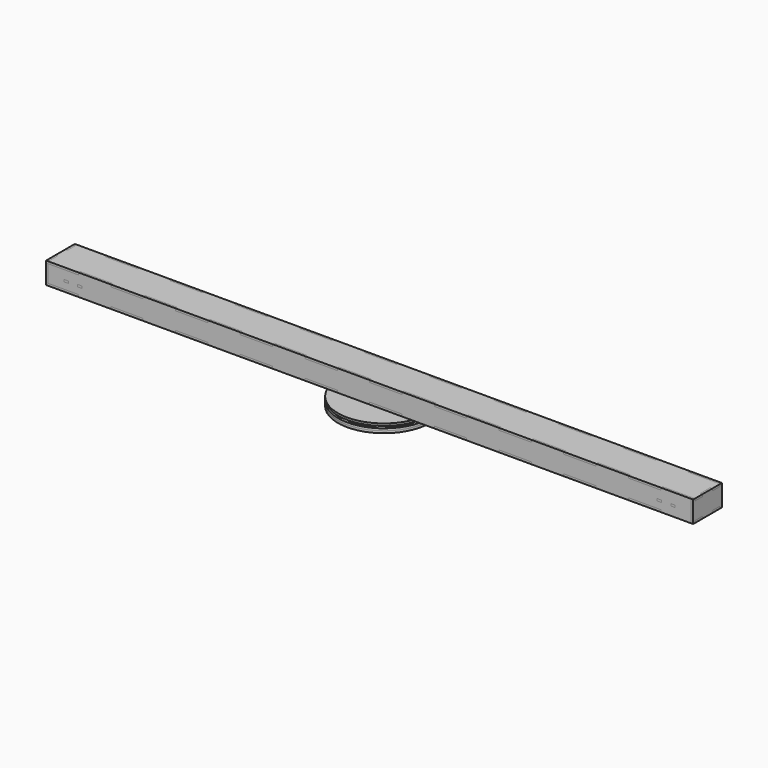
from build123d import *

# Parameters (mm, degrees)
F3_R         = 64
F3_R_2       = 20.5
F3_W         = 6
F3_H         = 6.5
F3_H_2       = 6
F3_R_3       = 1.5
F23_DEPTH    = 3
F5_R         = 20.5
F24_DEPTH    = 3
F6_R         = 1.6
F6_R_2       = 2.5
F6_R_3       = 12.5
F6_W         = 750
F6_H         = 20
F6_W_2       = 3
F6_H_2       = 16.6666666667
F6_W_3       = 45
F6_H_3       = 3
F6_H_4       = 13.6666666667
F25_DEPTH    = 3
F8_W         = 900
F8_H         = 30
F26_DEPTH    = 3
F10_W        = 900
F10_H        = 30
F27_DEPTH    = 3
F12_W        = 50
F12_H        = 30
F28_DEPTH    = 3
F14_W        = 50
F14_H        = 30
F29_DEPTH    = 3
F16_W        = 3
F16_H        = 16.6666666667
F16_W_2      = 45
F16_H_2      = 3
F16_H_3      = 13.6666666667
F30_DEPTH    = 3
F31_DEPTH    = 3
F32_DEPTH    = 3
F33_DEPTH    = 3
F34_DEPTH    = 3
F35_DEPTH    = 3
F18_R        = 1.6
F36_DEPTH    = 3
F37_DEPTH    = 3
F37_FACE_R   = 1.6
F36_FACE_R   = 1.6
F38_DEPTH    = 3
F39_DEPTH    = 3
F21_R        = 64
F40_DEPTH    = 3
F23_FACE_R   = 64
F23_FACE_R_2 = 1.5
F41_DEPTH    = 3
F42_DEPTH    = 3


# Not quite as in the source:
# - a feature names something its author has since deleted; it is built from what else it names


with BuildPart() as f23:
    # F3 (on Top) → F23 (new body)
    with BuildSketch(Plane.XY):
        Circle(F3_R)
        Circle(F3_R_2, mode=Mode.SUBTRACT)
        Circle(F3_R_2)
        with BuildLine():
            ThreePointArc((14.6969384567, 3), (14.9240422951, 1.5076344301), (15, 0))
            ThreePointArc((15, 0), (14.9240422951, -1.5076344301), (14.6969384567, -3))
            ThreePointArc((14.6969384567, -3), (10.6066017178, -10.6066017178), (3, -14.6969384567))
            ThreePointArc((3, -14.6969384567), (0, -15), (-3, -14.6969384567))
            ThreePointArc((-3, -14.6969384567), (-10.6066017178, -10.6066017178), (-14.6969384567, -3))
            ThreePointArc((-14.6969384567, -3), (-15, 0), (-14.6969384567, 3))
            ThreePointArc((-14.6969384567, 3), (-10.6066017178, 10.6066017178), (-3, 14.6969384567))
            ThreePointArc((-3, 14.6969384567), (0, 15), (3, 14.6969384567))
            ThreePointArc((3, 14.6969384567), (10.6066017178, 10.6066017178), (14.6969384567, 3))
        make_face(mode=Mode.SUBTRACT)
        with Locations((0, -6.25)):
            Rectangle(F3_W, F3_H)
        with BuildLine():
            ThreePointArc((-3, -14.6969384567), (0, -15), (3, -14.6969384567))
            Line((3, -14.6969384567), (3, -9.5))
            Line((3, -9.5), (-3, -9.5))
            Line((-3, -9.5), (-3, -14.6969384567))
        make_face()
        with Locations((0, 6.25)):
            Rectangle(F3_W, F3_H)
        with BuildLine():
            Line((3, 9.5), (3, 14.6969384567))
            ThreePointArc((3, 14.6969384567), (0, 15), (-3, 14.6969384567))
            Line((-3, 14.6969384567), (-3, 9.5))
            Line((-3, 9.5), (3, 9.5))
        make_face()
        Rectangle(F3_W, F3_H_2)
        Circle(F3_R_3, mode=Mode.SUBTRACT)
    extrude(amount=-F23_DEPTH)


with BuildPart() as f24:
    # F5 (on offset) → F24 (new body)
    with BuildSketch(Plane.XY.offset(3)):
        Circle(F5_R)
        with BuildLine():
            ThreePointArc((14.6969384567, 3), (14.9240422951, 1.5076344301), (15, 0))
            ThreePointArc((15, 0), (14.9240422951, -1.5076344301), (14.6969384567, -3))
            ThreePointArc((14.6969384567, -3), (10.6066017178, -10.6066017178), (3, -14.6969384567))
            ThreePointArc((3, -14.6969384567), (0, -15), (-3, -14.6969384567))
            ThreePointArc((-3, -14.6969384567), (-10.6066017178, -10.6066017178), (-14.6969384567, -3))
            ThreePointArc((-14.6969384567, -3), (-15, 0), (-14.6969384567, 3))
            ThreePointArc((-14.6969384567, 3), (-10.6066017178, 10.6066017178), (-3, 14.6969384567))
            ThreePointArc((-3, 14.6969384567), (0, 15), (3, 14.6969384567))
            ThreePointArc((3, 14.6969384567), (10.6066017178, 10.6066017178), (14.6969384567, 3))
        make_face(mode=Mode.SUBTRACT)
        with BuildLine():
            ThreePointArc((-3, -14.6969384567), (0, -15), (3, -14.6969384567))
            Line((3, -14.6969384567), (3, -3))
            Line((3, -3), (-3, -3))
            Line((-3, -3), (-3, -14.6969384567))
        make_face()
        with BuildLine():
            ThreePointArc((14.6969384567, -3), (14.9240422951, -1.5076344301), (15, 0))
            ThreePointArc((15, 0), (14.9240422951, 1.5076344301), (14.6969384567, 3))
            Line((14.6969384567, 3), (3, 3))
            Line((3, 3), (-3, 3))
            Line((-3, 3), (-14.6969384567, 3))
            ThreePointArc((-14.6969384567, 3), (-15, 0), (-14.6969384567, -3))
            Line((-14.6969384567, -3), (-3, -3))
            Line((-3, -3), (3, -3))
            Line((3, -3), (14.6969384567, -3))
        make_face()
        with BuildLine():
            Line((3, 3), (3, 14.6969384567))
            ThreePointArc((3, 14.6969384567), (0, 15), (-3, 14.6969384567))
            Line((-3, 14.6969384567), (-3, 3))
            Line((-3, 3), (3, 3))
        make_face()
    extrude(amount=F24_DEPTH)


with BuildPart() as f25:
    # F6 (on offset) → F25 (new body)
    with BuildSketch(Plane.XY.offset(3)):
        Polygon((-360, 22), (-405, 22), (-447, 22), (-447, 8.3333333333), (-447, -8.3333333333), (-447, -22), (-405, -22), (-360, -22), (-315, -22), (-270, -22), (-225, -22), (-180, -22), (-135, -22), (-90, -22), (-45, -22), (0, -22), (45, -22), (90, -22), (135, -22), (180, -22), (225, -22), (270, -22), (315, -22), (360, -22), (405, -22), (447, -22), (447, -8.3333333333), (447, 8.3333333333), (447, 22), (405, 22), (360, 22), (315, 22), (270, 22), (225, 22), (180, 22), (135, 22), (90, 22), (45, 22), (0, 22), (-45, 22), (-90, 22), (-135, 22), (-180, 22), (-225, 22), (-270, 22), (-315, 22), align=None)
        with Locations((-386.593101397, -10.4)):
            Circle(F6_R, mode=Mode.SUBTRACT)
        with Locations((386.593101397, -10.4)):
            Circle(F6_R, mode=Mode.SUBTRACT)
        with Locations((-435.5, 0)):
            Circle(F6_R_2, mode=Mode.SUBTRACT)
        with Locations((-412.5, 0)):
            Circle(F6_R_3, mode=Mode.SUBTRACT)
        with Locations((-386.593101397, 10.4)):
            Circle(F6_R, mode=Mode.SUBTRACT)
        Rectangle(F6_W, F6_H, mode=Mode.SUBTRACT)
        with Locations((412.5, 0)):
            Circle(F6_R_3, mode=Mode.SUBTRACT)
        with Locations((435.5, 0)):
            Circle(F6_R_2, mode=Mode.SUBTRACT)
        with Locations((386.593101397, 10.4)):
            Circle(F6_R, mode=Mode.SUBTRACT)
        with Locations((-448.5, 0)):
            Rectangle(F6_W_2, F6_H_2)
        Polygon((-405, 25), (-450, 25), (-450, 22), (-447, 22), (-405, 22), align=None)
        Polygon((-447, -22), (-450, -22), (-450, -25), (-405, -25), (-405, -22), align=None)
        with Locations((-337.5, -23.5)):
            Rectangle(F6_W_3, F6_H_3)
        with Locations((-337.5, 23.5)):
            Rectangle(F6_W_3, F6_H_3)
        with Locations((-247.5, 23.5)):
            Rectangle(F6_W_3, F6_H_3)
        with Locations((-247.5, -23.5)):
            Rectangle(F6_W_3, F6_H_3)
        with Locations((-157.5, 23.5)):
            Rectangle(F6_W_3, F6_H_3)
        with Locations((-67.5, 23.5)):
            Rectangle(F6_W_3, F6_H_3)
        with Locations((-67.5, -23.5)):
            Rectangle(F6_W_3, F6_H_3)
        with Locations((-157.5, -23.5)):
            Rectangle(F6_W_3, F6_H_3)
        with Locations((22.5, 23.5)):
            Rectangle(F6_W_3, F6_H_3)
        with Locations((22.5, -23.5)):
            Rectangle(F6_W_3, F6_H_3)
        with Locations((112.5, -23.5)):
            Rectangle(F6_W_3, F6_H_3)
        with Locations((112.5, 23.5)):
            Rectangle(F6_W_3, F6_H_3)
        with Locations((202.5, 23.5)):
            Rectangle(F6_W_3, F6_H_3)
        with Locations((202.5, -23.5)):
            Rectangle(F6_W_3, F6_H_3)
        with Locations((292.5, -23.5)):
            Rectangle(F6_W_3, F6_H_3)
        with Locations((292.5, 23.5)):
            Rectangle(F6_W_3, F6_H_3)
        with Locations((382.5, 23.5)):
            Rectangle(F6_W_3, F6_H_3)
        with Locations((382.5, -23.5)):
            Rectangle(F6_W_3, F6_H_3)
        with Locations((448.5, -15.1666666667)):
            Rectangle(F6_W_2, F6_H_4)
        with Locations((448.5, 15.1666666667)):
            Rectangle(F6_W_2, F6_H_4)
        with Locations((412.5, 0)):
            Circle(F6_R_3)
        with Locations((412.5, 0)):
            Circle(F6_R, mode=Mode.SUBTRACT)
        with Locations((-412.5, 0)):
            Circle(F6_R_3)
        with Locations((-412.5, 0)):
            Circle(F6_R, mode=Mode.SUBTRACT)
    extrude(amount=-F25_DEPTH)


with BuildPart() as f26:
    # F8 (on line) → F26 (new body)
    with BuildSketch(Plane(origin=(0, -25, 0), x_dir=(-1, 0, 0), z_dir=(0, 1, 0))):
        with Locations((0, 15)):
            Rectangle(F8_W, F8_H)
    extrude(amount=F26_DEPTH)


with BuildPart() as f27:
    # F10 (on line) → F27 (new body)
    with BuildSketch(Plane(origin=(0, 25, 0), x_dir=(-1, 0, 0), z_dir=(0, 1, 0))):
        with Locations((0, 15)):
            Rectangle(F10_W, F10_H)
    extrude(amount=-F27_DEPTH)


with BuildPart() as f28:
    # F12 (on line) → F28 (new body)
    with BuildSketch(Plane.YZ.offset(450)):
        with Locations((0, 15)):
            Rectangle(F12_W, F12_H)
    extrude(amount=-F28_DEPTH)


with BuildPart() as f29:
    # F14 (on line) → F29 (new body)
    with BuildSketch(Plane.YZ.offset(-450)):
        with Locations((0, 15)):
            Rectangle(F14_W, F14_H)
    extrude(amount=F29_DEPTH)


with BuildPart() as f30:
    # F16 (on line) → F30 (new body)
    with BuildSketch(Plane.XY.offset(30)):
        with Locations((-448.5, 0)):
            Rectangle(F16_W, F16_H)
        Polygon((-405, 25), (-450, 25), (-450, 22), (-447, 22), (-405, 22), align=None)
        Polygon((-447, -22), (-450, -22), (-450, -25), (-405, -25), (-405, -22), align=None)
        with Locations((-337.5, 23.5)):
            Rectangle(F16_W_2, F16_H_2)
        with Locations((-337.5, -23.5)):
            Rectangle(F16_W_2, F16_H_2)
        with Locations((-247.5, 23.5)):
            Rectangle(F16_W_2, F16_H_2)
        with Locations((-247.5, -23.5)):
            Rectangle(F16_W_2, F16_H_2)
        with Locations((-157.5, 23.5)):
            Rectangle(F16_W_2, F16_H_2)
        with Locations((-157.5, -23.5)):
            Rectangle(F16_W_2, F16_H_2)
        with Locations((-67.5, 23.5)):
            Rectangle(F16_W_2, F16_H_2)
        with Locations((-67.5, -23.5)):
            Rectangle(F16_W_2, F16_H_2)
        with Locations((22.5, 23.5)):
            Rectangle(F16_W_2, F16_H_2)
        with Locations((22.5, -23.5)):
            Rectangle(F16_W_2, F16_H_2)
        with Locations((112.5, 23.5)):
            Rectangle(F16_W_2, F16_H_2)
        with Locations((112.5, -23.5)):
            Rectangle(F16_W_2, F16_H_2)
        with Locations((202.5, -23.5)):
            Rectangle(F16_W_2, F16_H_2)
        with Locations((202.5, 23.5)):
            Rectangle(F16_W_2, F16_H_2)
        with Locations((292.5, 23.5)):
            Rectangle(F16_W_2, F16_H_2)
        with Locations((292.5, -23.5)):
            Rectangle(F16_W_2, F16_H_2)
        with Locations((382.5, -23.5)):
            Rectangle(F16_W_2, F16_H_2)
        with Locations((382.5, 23.5)):
            Rectangle(F16_W_2, F16_H_2)
        with Locations((448.5, 15.1666666667)):
            Rectangle(F16_W, F16_H_3)
        with Locations((448.5, -15.1666666667)):
            Rectangle(F16_W, F16_H_3)
        Polygon((-360, 22), (-405, 22), (-447, 22), (-447, 8.3333333333), (-447, -8.3333333333), (-447, -22), (-405, -22), (-360, -22), (-315, -22), (-270, -22), (-225, -22), (-180, -22), (-135, -22), (-90, -22), (-45, -22), (0, -22), (45, -22), (90, -22), (135, -22), (180, -22), (225, -22), (270, -22), (315, -22), (360, -22), (405, -22), (447, -22), (447, -8.3333333333), (447, 8.3333333333), (447, 22), (405, 22), (360, 22), (315, 22), (270, 22), (225, 22), (180, 22), (135, 22), (90, 22), (45, 22), (0, 22), (-45, 22), (-90, 22), (-135, 22), (-180, 22), (-225, 22), (-270, 22), (-315, 22), align=None)
    extrude(amount=-F30_DEPTH)


with BuildPart() as f31_tool:
    # F31 (cut): a face of the model
    f31_faces = [f30.part.faces().sort_by_distance(p)[0] for p in [
        (-1.1003130336, 0, 30),
    ]]
    extrude(f31_faces, amount=-F31_DEPTH)


with BuildPart() as f26_1:
    add(f26.part)

    # F31: cut by f31_tool
    add(f31_tool.part, mode=Mode.SUBTRACT)


with BuildPart() as f27_1:
    add(f27.part)

    # F31: cut by f31_tool
    add(f31_tool.part, mode=Mode.SUBTRACT)


with BuildPart() as f28_1:
    add(f28.part)

    # F31: cut by f31_tool
    add(f31_tool.part, mode=Mode.SUBTRACT)


with BuildPart() as f29_1:
    add(f29.part)

    # F31: cut by f31_tool
    add(f31_tool.part, mode=Mode.SUBTRACT)


with BuildPart() as f32_tool:
    # F32 (cut): a face of the model
    f32_faces = [f25.part.faces().sort_by_distance(p)[0] for p in [
        (446.0986121811, 0, 0),
    ]]
    extrude(f32_faces, amount=-F32_DEPTH)


with BuildPart() as f26_2:
    add(f26_1.part)

    # F32: cut by f32_tool
    add(f32_tool.part, mode=Mode.SUBTRACT)


with BuildPart() as f27_2:
    add(f27_1.part)

    # F32: cut by f32_tool
    add(f32_tool.part, mode=Mode.SUBTRACT)


with BuildPart() as f28_2:
    add(f28_1.part)

    # F32: cut by f32_tool
    add(f32_tool.part, mode=Mode.SUBTRACT)


with BuildPart() as f29_2:
    add(f29_1.part)

    # F32: cut by f32_tool
    add(f32_tool.part, mode=Mode.SUBTRACT)


with BuildPart() as f33_tool:
    # F33 (cut): a face of the model
    f33_faces = [f29_2.part.faces().sort_by_distance(p)[0] for p in [
        (-450, 0, 15),
    ]]
    extrude(f33_faces, amount=-F33_DEPTH)


with BuildPart() as f26_3:
    add(f26_2.part)

    # F33: cut by f33_tool
    add(f33_tool.part, mode=Mode.SUBTRACT)


with BuildPart() as f27_3:
    add(f27_2.part)

    # F33: cut by f33_tool
    add(f33_tool.part, mode=Mode.SUBTRACT)


with BuildPart() as f34_tool:
    # F34 (cut): a face of the model
    f34_faces = [f28_2.part.faces().sort_by_distance(p)[0] for p in [
        (450, 0, 15),
    ]]
    extrude(f34_faces, amount=-F34_DEPTH)


with BuildPart() as f26_4:
    add(f26_3.part)

    # F34: cut by f34_tool
    add(f34_tool.part, mode=Mode.SUBTRACT)


with BuildPart() as f27_4:
    add(f27_3.part)

    # F34: cut by f34_tool
    add(f34_tool.part, mode=Mode.SUBTRACT)


with BuildPart() as f35:
    # F6 (on offset) → F35 (new body)
    with BuildSketch(Plane.XY.offset(3)):
        with Locations((-412.5, 0)):
            Circle(F6_R_3)
        with Locations((-412.5, 0)):
            Circle(F6_R, mode=Mode.SUBTRACT)
    extrude(amount=F35_DEPTH)


with BuildPart() as f36:
    # F18 (on offset) → F36 (new body)
    with BuildSketch(Plane.XY.offset(12)):
        Polygon((-419, 25), (-425, 25), (-425, 22), (-425, -25), (-419, -25), (-419, -22), (-406, -22), (-406, -25), (-400, -25), (-400, 22), (-400, 25), (-406, 25), (-406, 22), (-419, 22), align=None)
        with Locations((-412.5, 0)):
            Circle(F18_R, mode=Mode.SUBTRACT)
    extrude(amount=F36_DEPTH)


with BuildPart() as f37:
    # F18 (on offset) → F37 (new body)
    with BuildSketch(Plane.XY.offset(12)):
        Polygon((406, 25), (400, 25), (400, 22), (400, -25), (406, -25), (406, -22), (419, -22), (419, -25), (425, -25), (425, 22), (425, 25), (419, 25), (419, 22), (406, 22), align=None)
        with Locations((412.5, 0)):
            Circle(F18_R, mode=Mode.SUBTRACT)
    extrude(amount=F37_DEPTH)


with BuildPart() as f37b:
    # F18 (on offset) → F37, piece 2 (new body)
    with BuildSketch(Plane.XY.offset(12)):
        Polygon((-419, 25), (-425, 25), (-425, 22), (-425, -25), (-419, -25), (-419, -22), (-406, -22), (-406, -25), (-400, -25), (-400, 22), (-400, 25), (-406, 25), (-406, 22), (-419, 22), align=None)
        with Locations((-412.5, 0)):
            Circle(F18_R, mode=Mode.SUBTRACT)
    extrude(amount=F37_DEPTH)


with BuildPart() as f38_tool:
    # F37_face (on face) + F36_face (on face) → F38 (new body)
    with BuildSketch(Plane(origin=(412.5, 0, 15), x_dir=(1, 0, 0), z_dir=(0, 0, 1))):
        Polygon((-6.5, 25), (-12.5, 25), (-12.5, -25), (-6.5, -25), (-6.5, -22), (6.5, -22), (6.5, -25), (12.5, -25), (12.5, 25), (6.5, 25), (6.5, 22), (-6.5, 22), align=None)
        Circle(F37_FACE_R, mode=Mode.SUBTRACT)
    with BuildSketch(Plane(origin=(-412.5, 0, 15), x_dir=(1, 0, 0), z_dir=(0, 0, 1))):
        Polygon((-6.5, 25), (-12.5, 25), (-12.5, -25), (-6.5, -25), (-6.5, -22), (6.5, -22), (6.5, -25), (12.5, -25), (12.5, 25), (6.5, 25), (6.5, 22), (-6.5, 22), align=None)
        Circle(F36_FACE_R, mode=Mode.SUBTRACT)
    extrude(amount=-F38_DEPTH)


with BuildPart() as f26_5:
    add(f26_4.part)

    # F38: cut by f38_tool
    add(f38_tool.part, mode=Mode.SUBTRACT)


with BuildPart() as f27_5:
    add(f27_4.part)

    # F38: cut by f38_tool
    add(f38_tool.part, mode=Mode.SUBTRACT)


with BuildPart() as f39:
    # F3 (on Top) → F39 (new body)
    with BuildSketch(Plane.XY):
        with Locations((0, -6.25)):
            Rectangle(F3_W, F3_H)
        Rectangle(F3_W, F3_H_2)
        Circle(F3_R_3, mode=Mode.SUBTRACT)
        with Locations((0, 6.25)):
            Rectangle(F3_W, F3_H)
    extrude(amount=F39_DEPTH)


with BuildPart() as f40:
    # F21 (on offset) → F40 (new body)
    with BuildSketch(Plane.XY.offset(-9)):
        Circle(F21_R)
        with BuildLine():
            ThreePointArc((60.0732729337, 10.5925388377), (60.7678765836, 5.3165003076), (61, 0))
            ThreePointArc((61, 0), (60.7678765836, -5.3165003076), (60.0732729337, -10.5925388377))
            ThreePointArc((60.0732729337, -10.5925388377), (58.9214754036, -15.7879617513), (57.3212498679, -20.8632287429))
            ThreePointArc((57.3212498679, -20.8632287429), (55.2847750092, -25.7797139662), (52.8275496309, -30.5))
            ThreePointArc((52.8275496309, -30.5), (49.9682747016, -34.9881626174), (46.7287110303, -39.2100441909))
            ThreePointArc((46.7287110303, -39.2100441909), (43.1335136524, -43.1335136524), (39.2100441909, -46.7287110303))
            ThreePointArc((39.2100441909, -46.7287110303), (34.9881626174, -49.9682747016), (30.5, -52.8275496309))
            ThreePointArc((30.5, -52.8275496309), (25.7797139662, -55.2847750092), (20.8632287429, -57.3212498679))
            ThreePointArc((20.8632287429, -57.3212498679), (15.7879617513, -58.9214754036), (10.5925388377, -60.0732729337))
            ThreePointArc((10.5925388377, -60.0732729337), (5.3165003076, -60.7678765836), (0, -61))
            ThreePointArc((0, -61), (-5.3165003076, -60.7678765836), (-10.5925388377, -60.0732729337))
            ThreePointArc((-10.5925388377, -60.0732729337), (-15.7879617513, -58.9214754036), (-20.8632287429, -57.3212498679))
            ThreePointArc((-20.8632287429, -57.3212498679), (-25.7797139662, -55.2847750092), (-30.5, -52.8275496309))
            ThreePointArc((-30.5, -52.8275496309), (-34.9881626174, -49.9682747016), (-39.2100441909, -46.7287110303))
            ThreePointArc((-39.2100441909, -46.7287110303), (-43.1335136524, -43.1335136524), (-46.7287110303, -39.2100441909))
            ThreePointArc((-46.7287110303, -39.2100441909), (-49.9682747016, -34.9881626174), (-52.8275496309, -30.5))
            ThreePointArc((-52.8275496309, -30.5), (-55.2847750092, -25.7797139662), (-57.3212498679, -20.8632287429))
            ThreePointArc((-57.3212498679, -20.8632287429), (-58.9214754036, -15.7879617513), (-60.0732729337, -10.5925388377))
            ThreePointArc((-60.0732729337, -10.5925388377), (-60.7678765836, -5.3165003076), (-61, 0))
            ThreePointArc((-61, 0), (-60.7678765836, 5.3165003076), (-60.0732729337, 10.5925388377))
            ThreePointArc((-60.0732729337, 10.5925388377), (-58.9214754036, 15.7879617513), (-57.3212498679, 20.8632287429))
            ThreePointArc((-57.3212498679, 20.8632287429), (-55.2847750092, 25.7797139662), (-52.8275496309, 30.5))
            ThreePointArc((-52.8275496309, 30.5), (-49.9682747016, 34.9881626174), (-46.7287110303, 39.2100441909))
            ThreePointArc((-46.7287110303, 39.2100441909), (-43.1335136524, 43.1335136524), (-39.2100441909, 46.7287110303))
            ThreePointArc((-39.2100441909, 46.7287110303), (-34.9881626174, 49.9682747016), (-30.5, 52.8275496309))
            ThreePointArc((-30.5, 52.8275496309), (-25.7797139662, 55.2847750092), (-20.8632287429, 57.3212498679))
            ThreePointArc((-20.8632287429, 57.3212498679), (-15.7879617513, 58.9214754036), (-10.5925388377, 60.0732729337))
            ThreePointArc((-10.5925388377, 60.0732729337), (-5.3165003076, 60.7678765836), (0, 61))
            ThreePointArc((0, 61), (5.3165003076, 60.7678765836), (10.5925388377, 60.0732729337))
            ThreePointArc((10.5925388377, 60.0732729337), (15.7879617513, 58.9214754036), (20.8632287429, 57.3212498679))
            ThreePointArc((20.8632287429, 57.3212498679), (25.7797139662, 55.2847750092), (30.5, 52.8275496309))
            ThreePointArc((30.5, 52.8275496309), (34.9881626174, 49.9682747016), (39.2100441909, 46.7287110303))
            ThreePointArc((39.2100441909, 46.7287110303), (43.1335136524, 43.1335136524), (46.7287110303, 39.2100441909))
            ThreePointArc((46.7287110303, 39.2100441909), (49.9682747016, 34.9881626174), (52.8275496309, 30.5))
            ThreePointArc((52.8275496309, 30.5), (55.2847750092, 25.7797139662), (57.3212498679, 20.8632287429))
            ThreePointArc((57.3212498679, 20.8632287429), (58.9214754036, 15.7879617513), (60.0732729337, 10.5925388377))
        make_face(mode=Mode.SUBTRACT)
    extrude(amount=F40_DEPTH)

    # F21 (on offset) + F23_face (on face) → F41 (join)
    with BuildSketch(Plane.XY.offset(-9)):
        with BuildLine():
            ThreePointArc((19.8371683129, -54.5021720056), (24.511859181, -52.5658516481), (29, -50.2294734195))
            Line((29, -50.2294734195), (27.5, -47.6313972081))
            ThreePointArc((27.5, -47.6313972081), (23.2440043957, -49.846928287), (18.8111078829, -51.6830941432))
            Line((18.8111078829, -51.6830941432), (19.8371683129, -54.5021720056))
        make_face()
        with BuildLine():
            ThreePointArc((30.5, -52.8275496309), (34.9881626174, -49.9682747016), (39.2100441909, -46.7287110303))
            Line((39.2100441909, -46.7287110303), (37.2816813618, -44.4305777009))
            ThreePointArc((37.2816813618, -44.4305777009), (33.2674333084, -47.5108185688), (29, -50.2294734195))
            Line((29, -50.2294734195), (30.5, -52.8275496309))
        make_face()
        with BuildLine():
            ThreePointArc((29, -50.2294734195), (33.2674333084, -47.5108185688), (37.2816813618, -44.4305777009))
            Line((37.2816813618, -44.4305777009), (35.3533185328, -42.1324443715))
            ThreePointArc((35.3533185328, -42.1324443715), (31.5467039993, -45.0533624359), (27.5, -47.6313972081))
            Line((27.5, -47.6313972081), (29, -50.2294734195))
        make_face()
        with BuildLine():
            Line((0, -58), (0, -55))
            ThreePointArc((0, -55), (-4.7935658511, -54.790708395), (-9.5506497717, -54.1644264157))
            Line((-9.5506497717, -54.1644264157), (-10.0715943047, -57.1188496747))
            ThreePointArc((-10.0715943047, -57.1188496747), (-5.0550330794, -57.7792924893), (0, -58))
        make_face()
        with BuildLine():
            ThreePointArc((-10.5925388377, -60.0732729337), (-5.3165003076, -60.7678765836), (0, -61))
            Line((0, -61), (0, -58))
            ThreePointArc((0, -58), (-5.0550330794, -57.7792924893), (-10.0715943047, -57.1188496747))
            Line((-10.0715943047, -57.1188496747), (-10.5925388377, -60.0732729337))
        make_face()
        with BuildLine():
            ThreePointArc((-9.5506497717, -54.1644264157), (-14.2350474806, -53.1259204459), (-18.8111078829, -51.6830941432))
            Line((-18.8111078829, -51.6830941432), (-19.8371683129, -54.5021720056))
            ThreePointArc((-19.8371683129, -54.5021720056), (-15.0115046159, -56.0236979248), (-10.0715943047, -57.1188496747))
            Line((-10.0715943047, -57.1188496747), (-9.5506497717, -54.1644264157))
        make_face()
        with BuildLine():
            ThreePointArc((50.2294734195, -29), (52.5658516481, -24.511859181), (54.5021720056, -19.8371683129))
            Line((54.5021720056, -19.8371683129), (51.6830941432, -18.8111078829))
            ThreePointArc((51.6830941432, -18.8111078829), (49.846928287, -23.2440043957), (47.6313972081, -27.5))
            Line((47.6313972081, -27.5), (50.2294734195, -29))
        make_face()
        with BuildLine():
            ThreePointArc((54.5021720056, -19.8371683129), (56.0236979248, -15.0115046159), (57.1188496747, -10.0715943047))
            Line((57.1188496747, -10.0715943047), (54.1644264157, -9.5506497717))
            ThreePointArc((54.1644264157, -9.5506497717), (53.1259204459, -14.2350474806), (51.6830941432, -18.8111078829))
            Line((51.6830941432, -18.8111078829), (54.5021720056, -19.8371683129))
        make_face()
        with BuildLine():
            ThreePointArc((57.3212498679, -20.8632287429), (58.9214754036, -15.7879617513), (60.0732729337, -10.5925388377))
            Line((60.0732729337, -10.5925388377), (57.1188496747, -10.0715943047))
            ThreePointArc((57.1188496747, -10.0715943047), (56.0236979248, -15.0115046159), (54.5021720056, -19.8371683129))
            Line((54.5021720056, -19.8371683129), (57.3212498679, -20.8632287429))
        make_face()
        with BuildLine():
            Line((54.1644264157, 9.5506497717), (57.1188496747, 10.0715943047))
            ThreePointArc((57.1188496747, 10.0715943047), (56.0236979248, 15.0115046159), (54.5021720056, 19.8371683129))
            Line((54.5021720056, 19.8371683129), (51.6830941432, 18.8111078829))
            ThreePointArc((51.6830941432, 18.8111078829), (53.1259204459, 14.2350474806), (54.1644264157, 9.5506497717))
        make_face()
        with BuildLine():
            Line((51.6830941432, 18.8111078829), (54.5021720056, 19.8371683129))
            ThreePointArc((54.5021720056, 19.8371683129), (52.5658516481, 24.511859181), (50.2294734195, 29))
            Line((50.2294734195, 29), (47.6313972081, 27.5))
            ThreePointArc((47.6313972081, 27.5), (49.846928287, 23.2440043957), (51.6830941432, 18.8111078829))
        make_face()
        with BuildLine():
            Line((54.5021720056, 19.8371683129), (57.3212498679, 20.8632287429))
            ThreePointArc((57.3212498679, 20.8632287429), (55.2847750092, 25.7797139662), (52.8275496309, 30.5))
            Line((52.8275496309, 30.5), (50.2294734195, 29))
            ThreePointArc((50.2294734195, 29), (52.5658516481, 24.511859181), (54.5021720056, 19.8371683129))
        make_face()
        with BuildLine():
            Line((35.3533185328, 42.1324443715), (37.2816813618, 44.4305777009))
            ThreePointArc((37.2816813618, 44.4305777009), (33.2674333084, 47.5108185688), (29, 50.2294734195))
            Line((29, 50.2294734195), (27.5, 47.6313972081))
            ThreePointArc((27.5, 47.6313972081), (31.5467039993, 45.0533624359), (35.3533185328, 42.1324443715))
        make_face()
        with BuildLine():
            Line((27.5, 47.6313972081), (29, 50.2294734195))
            ThreePointArc((29, 50.2294734195), (24.511859181, 52.5658516481), (19.8371683129, 54.5021720056))
            Line((19.8371683129, 54.5021720056), (18.8111078829, 51.6830941432))
            ThreePointArc((18.8111078829, 51.6830941432), (23.2440043957, 49.846928287), (27.5, 47.6313972081))
        make_face()
        with BuildLine():
            Line((29, 50.2294734195), (30.5, 52.8275496309))
            ThreePointArc((30.5, 52.8275496309), (25.7797139662, 55.2847750092), (20.8632287429, 57.3212498679))
            Line((20.8632287429, 57.3212498679), (19.8371683129, 54.5021720056))
            ThreePointArc((19.8371683129, 54.5021720056), (24.511859181, 52.5658516481), (29, 50.2294734195))
        make_face()
        with BuildLine():
            ThreePointArc((-9.5506497717, 54.1644264157), (-4.7935658511, 54.790708395), (0, 55))
            Line((0, 55), (0, 58))
            ThreePointArc((0, 58), (-5.0550330794, 57.7792924893), (-10.0715943047, 57.1188496747))
            Line((-10.0715943047, 57.1188496747), (-9.5506497717, 54.1644264157))
        make_face()
        with BuildLine():
            ThreePointArc((-18.8111078829, 51.6830941432), (-14.2350474806, 53.1259204459), (-9.5506497717, 54.1644264157))
            Line((-9.5506497717, 54.1644264157), (-10.0715943047, 57.1188496747))
            ThreePointArc((-10.0715943047, 57.1188496747), (-15.0115046159, 56.0236979248), (-19.8371683129, 54.5021720056))
            Line((-19.8371683129, 54.5021720056), (-18.8111078829, 51.6830941432))
        make_face()
        with BuildLine():
            ThreePointArc((-19.8371683129, 54.5021720056), (-15.0115046159, 56.0236979248), (-10.0715943047, 57.1188496747))
            Line((-10.0715943047, 57.1188496747), (-10.5925388377, 60.0732729337))
            ThreePointArc((-10.5925388377, 60.0732729337), (-15.7879617513, 58.9214754036), (-20.8632287429, 57.3212498679))
            Line((-20.8632287429, 57.3212498679), (-19.8371683129, 54.5021720056))
        make_face()
        with BuildLine():
            ThreePointArc((-47.6313972081, 27.5), (-45.0533624359, 31.5467039993), (-42.1324443715, 35.3533185328))
            Line((-42.1324443715, 35.3533185328), (-44.4305777009, 37.2816813618))
            ThreePointArc((-44.4305777009, 37.2816813618), (-47.5108185688, 33.2674333084), (-50.2294734195, 29))
            Line((-50.2294734195, 29), (-47.6313972081, 27.5))
        make_face()
        with BuildLine():
            ThreePointArc((-50.2294734195, 29), (-47.5108185688, 33.2674333084), (-44.4305777009, 37.2816813618))
            Line((-44.4305777009, 37.2816813618), (-46.7287110303, 39.2100441909))
            ThreePointArc((-46.7287110303, 39.2100441909), (-49.9682747016, 34.9881626174), (-52.8275496309, 30.5))
            Line((-52.8275496309, 30.5), (-50.2294734195, 29))
        make_face()
        with BuildLine():
            ThreePointArc((-42.1324443715, 35.3533185328), (-38.8908729653, 38.8908729653), (-35.3533185328, 42.1324443715))
            Line((-35.3533185328, 42.1324443715), (-37.2816813618, 44.4305777009))
            ThreePointArc((-37.2816813618, 44.4305777009), (-41.0121933088, 41.0121933088), (-44.4305777009, 37.2816813618))
            Line((-44.4305777009, 37.2816813618), (-42.1324443715, 35.3533185328))
        make_face()
        with BuildLine():
            ThreePointArc((-54.1644264157, -9.5506497717), (-54.790708395, -4.7935658511), (-55, 0))
            Line((-55, 0), (-58, 0))
            ThreePointArc((-58, 0), (-57.7792924893, -5.0550330794), (-57.1188496747, -10.0715943047))
            Line((-57.1188496747, -10.0715943047), (-54.1644264157, -9.5506497717))
        make_face()
        with BuildLine():
            ThreePointArc((-55, 0), (-54.790708395, 4.7935658511), (-54.1644264157, 9.5506497717))
            Line((-54.1644264157, 9.5506497717), (-57.1188496747, 10.0715943047))
            ThreePointArc((-57.1188496747, 10.0715943047), (-57.7792924893, 5.0550330794), (-58, 0))
            Line((-58, 0), (-55, 0))
        make_face()
        with BuildLine():
            ThreePointArc((-57.1188496747, -10.0715943047), (-57.7792924893, -5.0550330794), (-58, 0))
            Line((-58, 0), (-61, 0))
            ThreePointArc((-61, 0), (-60.7678765836, -5.3165003076), (-60.0732729337, -10.5925388377))
            Line((-60.0732729337, -10.5925388377), (-57.1188496747, -10.0715943047))
        make_face()
        with BuildLine():
            ThreePointArc((-35.3533185328, -42.1324443715), (-38.8908729653, -38.8908729653), (-42.1324443715, -35.3533185328))
            Line((-42.1324443715, -35.3533185328), (-44.4305777009, -37.2816813618))
            ThreePointArc((-44.4305777009, -37.2816813618), (-41.0121933088, -41.0121933088), (-37.2816813618, -44.4305777009))
            Line((-37.2816813618, -44.4305777009), (-35.3533185328, -42.1324443715))
        make_face()
        with BuildLine():
            ThreePointArc((-37.2816813618, -44.4305777009), (-41.0121933088, -41.0121933088), (-44.4305777009, -37.2816813618))
            Line((-44.4305777009, -37.2816813618), (-46.7287110303, -39.2100441909))
            ThreePointArc((-46.7287110303, -39.2100441909), (-43.1335136524, -43.1335136524), (-39.2100441909, -46.7287110303))
            Line((-39.2100441909, -46.7287110303), (-37.2816813618, -44.4305777009))
        make_face()
        with BuildLine():
            ThreePointArc((-42.1324443715, -35.3533185328), (-45.0533624359, -31.5467039993), (-47.6313972081, -27.5))
            Line((-47.6313972081, -27.5), (-50.2294734195, -29))
            ThreePointArc((-50.2294734195, -29), (-47.5108185688, -33.2674333084), (-44.4305777009, -37.2816813618))
            Line((-44.4305777009, -37.2816813618), (-42.1324443715, -35.3533185328))
        make_face()
    with BuildSketch(Plane(origin=(0, 0, -3), x_dir=(1, 0, 0), z_dir=(0, 0, -1))):
        Circle(F23_FACE_R)
        with BuildLine():
            Line((3, -14.6969384567), (3, 14.6969384567))
            ThreePointArc((3, 14.6969384567), (15, 0), (3, -14.6969384567))
        make_face(mode=Mode.SUBTRACT)
        with BuildLine():
            ThreePointArc((-3, -14.6969384567), (-15, 0), (-3, 14.6969384567))
            Line((-3, 14.6969384567), (-3, -14.6969384567))
        make_face(mode=Mode.SUBTRACT)
        Circle(F23_FACE_R_2, mode=Mode.SUBTRACT)
    extrude(amount=F41_DEPTH, dir=(0, 0, 1))


with BuildPart() as f42:
    # F21 (on offset) → F42 (new body)
    with BuildSketch(Plane.XY.offset(-9)):
        Circle(F21_R)
        with BuildLine():
            ThreePointArc((60.0732729337, 10.5925388377), (60.7678765836, 5.3165003076), (61, 0))
            ThreePointArc((61, 0), (60.7678765836, -5.3165003076), (60.0732729337, -10.5925388377))
            ThreePointArc((60.0732729337, -10.5925388377), (58.9214754036, -15.7879617513), (57.3212498679, -20.8632287429))
            ThreePointArc((57.3212498679, -20.8632287429), (55.2847750092, -25.7797139662), (52.8275496309, -30.5))
            ThreePointArc((52.8275496309, -30.5), (49.9682747016, -34.9881626174), (46.7287110303, -39.2100441909))
            ThreePointArc((46.7287110303, -39.2100441909), (43.1335136524, -43.1335136524), (39.2100441909, -46.7287110303))
            ThreePointArc((39.2100441909, -46.7287110303), (34.9881626174, -49.9682747016), (30.5, -52.8275496309))
            ThreePointArc((30.5, -52.8275496309), (25.7797139662, -55.2847750092), (20.8632287429, -57.3212498679))
            ThreePointArc((20.8632287429, -57.3212498679), (15.7879617513, -58.9214754036), (10.5925388377, -60.0732729337))
            ThreePointArc((10.5925388377, -60.0732729337), (5.3165003076, -60.7678765836), (0, -61))
            ThreePointArc((0, -61), (-5.3165003076, -60.7678765836), (-10.5925388377, -60.0732729337))
            ThreePointArc((-10.5925388377, -60.0732729337), (-15.7879617513, -58.9214754036), (-20.8632287429, -57.3212498679))
            ThreePointArc((-20.8632287429, -57.3212498679), (-25.7797139662, -55.2847750092), (-30.5, -52.8275496309))
            ThreePointArc((-30.5, -52.8275496309), (-34.9881626174, -49.9682747016), (-39.2100441909, -46.7287110303))
            ThreePointArc((-39.2100441909, -46.7287110303), (-43.1335136524, -43.1335136524), (-46.7287110303, -39.2100441909))
            ThreePointArc((-46.7287110303, -39.2100441909), (-49.9682747016, -34.9881626174), (-52.8275496309, -30.5))
            ThreePointArc((-52.8275496309, -30.5), (-55.2847750092, -25.7797139662), (-57.3212498679, -20.8632287429))
            ThreePointArc((-57.3212498679, -20.8632287429), (-58.9214754036, -15.7879617513), (-60.0732729337, -10.5925388377))
            ThreePointArc((-60.0732729337, -10.5925388377), (-60.7678765836, -5.3165003076), (-61, 0))
            ThreePointArc((-61, 0), (-60.7678765836, 5.3165003076), (-60.0732729337, 10.5925388377))
            ThreePointArc((-60.0732729337, 10.5925388377), (-58.9214754036, 15.7879617513), (-57.3212498679, 20.8632287429))
            ThreePointArc((-57.3212498679, 20.8632287429), (-55.2847750092, 25.7797139662), (-52.8275496309, 30.5))
            ThreePointArc((-52.8275496309, 30.5), (-49.9682747016, 34.9881626174), (-46.7287110303, 39.2100441909))
            ThreePointArc((-46.7287110303, 39.2100441909), (-43.1335136524, 43.1335136524), (-39.2100441909, 46.7287110303))
            ThreePointArc((-39.2100441909, 46.7287110303), (-34.9881626174, 49.9682747016), (-30.5, 52.8275496309))
            ThreePointArc((-30.5, 52.8275496309), (-25.7797139662, 55.2847750092), (-20.8632287429, 57.3212498679))
            ThreePointArc((-20.8632287429, 57.3212498679), (-15.7879617513, 58.9214754036), (-10.5925388377, 60.0732729337))
            ThreePointArc((-10.5925388377, 60.0732729337), (-5.3165003076, 60.7678765836), (0, 61))
            ThreePointArc((0, 61), (5.3165003076, 60.7678765836), (10.5925388377, 60.0732729337))
            ThreePointArc((10.5925388377, 60.0732729337), (15.7879617513, 58.9214754036), (20.8632287429, 57.3212498679))
            ThreePointArc((20.8632287429, 57.3212498679), (25.7797139662, 55.2847750092), (30.5, 52.8275496309))
            ThreePointArc((30.5, 52.8275496309), (34.9881626174, 49.9682747016), (39.2100441909, 46.7287110303))
            ThreePointArc((39.2100441909, 46.7287110303), (43.1335136524, 43.1335136524), (46.7287110303, 39.2100441909))
            ThreePointArc((46.7287110303, 39.2100441909), (49.9682747016, 34.9881626174), (52.8275496309, 30.5))
            ThreePointArc((52.8275496309, 30.5), (55.2847750092, 25.7797139662), (57.3212498679, 20.8632287429))
            ThreePointArc((57.3212498679, 20.8632287429), (58.9214754036, 15.7879617513), (60.0732729337, 10.5925388377))
        make_face(mode=Mode.SUBTRACT)
        with BuildLine():
            Line((0, 58), (0, 61))
            ThreePointArc((0, 61), (-5.3165003076, 60.7678765836), (-10.5925388377, 60.0732729337))
            Line((-10.5925388377, 60.0732729337), (-10.0715943047, 57.1188496747))
            ThreePointArc((-10.0715943047, 57.1188496747), (-5.0550330794, 57.7792924893), (0, 58))
        make_face()
        with BuildLine():
            ThreePointArc((-19.8371683129, 54.5021720056), (-15.0115046159, 56.0236979248), (-10.0715943047, 57.1188496747))
            Line((-10.0715943047, 57.1188496747), (-10.5925388377, 60.0732729337))
            ThreePointArc((-10.5925388377, 60.0732729337), (-15.7879617513, 58.9214754036), (-20.8632287429, 57.3212498679))
            Line((-20.8632287429, 57.3212498679), (-19.8371683129, 54.5021720056))
        make_face()
        with BuildLine():
            ThreePointArc((-44.4305777009, 37.2816813618), (-41.0121933088, 41.0121933088), (-37.2816813618, 44.4305777009))
            Line((-37.2816813618, 44.4305777009), (-39.2100441909, 46.7287110303))
            ThreePointArc((-39.2100441909, 46.7287110303), (-43.1335136524, 43.1335136524), (-46.7287110303, 39.2100441909))
            Line((-46.7287110303, 39.2100441909), (-44.4305777009, 37.2816813618))
        make_face()
        with BuildLine():
            ThreePointArc((-50.2294734195, 29), (-47.5108185688, 33.2674333084), (-44.4305777009, 37.2816813618))
            Line((-44.4305777009, 37.2816813618), (-46.7287110303, 39.2100441909))
            ThreePointArc((-46.7287110303, 39.2100441909), (-49.9682747016, 34.9881626174), (-52.8275496309, 30.5))
            Line((-52.8275496309, 30.5), (-50.2294734195, 29))
        make_face()
        with BuildLine():
            ThreePointArc((-58, 0), (-57.7792924893, 5.0550330794), (-57.1188496747, 10.0715943047))
            Line((-57.1188496747, 10.0715943047), (-60.0732729337, 10.5925388377))
            ThreePointArc((-60.0732729337, 10.5925388377), (-60.7678765836, 5.3165003076), (-61, 0))
            Line((-61, 0), (-58, 0))
        make_face()
        with BuildLine():
            ThreePointArc((-57.1188496747, -10.0715943047), (-57.7792924893, -5.0550330794), (-58, 0))
            Line((-58, 0), (-61, 0))
            ThreePointArc((-61, 0), (-60.7678765836, -5.3165003076), (-60.0732729337, -10.5925388377))
            Line((-60.0732729337, -10.5925388377), (-57.1188496747, -10.0715943047))
        make_face()
        with BuildLine():
            ThreePointArc((-44.4305777009, -37.2816813618), (-47.5108185688, -33.2674333084), (-50.2294734195, -29))
            Line((-50.2294734195, -29), (-52.8275496309, -30.5))
            ThreePointArc((-52.8275496309, -30.5), (-49.9682747016, -34.9881626174), (-46.7287110303, -39.2100441909))
            Line((-46.7287110303, -39.2100441909), (-44.4305777009, -37.2816813618))
        make_face()
        with BuildLine():
            ThreePointArc((-37.2816813618, -44.4305777009), (-41.0121933088, -41.0121933088), (-44.4305777009, -37.2816813618))
            Line((-44.4305777009, -37.2816813618), (-46.7287110303, -39.2100441909))
            ThreePointArc((-46.7287110303, -39.2100441909), (-43.1335136524, -43.1335136524), (-39.2100441909, -46.7287110303))
            Line((-39.2100441909, -46.7287110303), (-37.2816813618, -44.4305777009))
        make_face()
        with BuildLine():
            ThreePointArc((-10.0715943047, -57.1188496747), (-15.0115046159, -56.0236979248), (-19.8371683129, -54.5021720056))
            Line((-19.8371683129, -54.5021720056), (-20.8632287429, -57.3212498679))
            ThreePointArc((-20.8632287429, -57.3212498679), (-15.7879617513, -58.9214754036), (-10.5925388377, -60.0732729337))
            Line((-10.5925388377, -60.0732729337), (-10.0715943047, -57.1188496747))
        make_face()
        with BuildLine():
            ThreePointArc((-10.5925388377, -60.0732729337), (-5.3165003076, -60.7678765836), (0, -61))
            Line((0, -61), (0, -58))
            ThreePointArc((0, -58), (-5.0550330794, -57.7792924893), (-10.0715943047, -57.1188496747))
            Line((-10.0715943047, -57.1188496747), (-10.5925388377, -60.0732729337))
        make_face()
        with BuildLine():
            ThreePointArc((20.8632287429, -57.3212498679), (25.7797139662, -55.2847750092), (30.5, -52.8275496309))
            Line((30.5, -52.8275496309), (29, -50.2294734195))
            ThreePointArc((29, -50.2294734195), (24.511859181, -52.5658516481), (19.8371683129, -54.5021720056))
            Line((19.8371683129, -54.5021720056), (20.8632287429, -57.3212498679))
        make_face()
        with BuildLine():
            ThreePointArc((30.5, -52.8275496309), (34.9881626174, -49.9682747016), (39.2100441909, -46.7287110303))
            Line((39.2100441909, -46.7287110303), (37.2816813618, -44.4305777009))
            ThreePointArc((37.2816813618, -44.4305777009), (33.2674333084, -47.5108185688), (29, -50.2294734195))
            Line((29, -50.2294734195), (30.5, -52.8275496309))
        make_face()
        with BuildLine():
            ThreePointArc((52.8275496309, -30.5), (55.2847750092, -25.7797139662), (57.3212498679, -20.8632287429))
            Line((57.3212498679, -20.8632287429), (54.5021720056, -19.8371683129))
            ThreePointArc((54.5021720056, -19.8371683129), (52.5658516481, -24.511859181), (50.2294734195, -29))
            Line((50.2294734195, -29), (52.8275496309, -30.5))
        make_face()
        with BuildLine():
            ThreePointArc((57.3212498679, -20.8632287429), (58.9214754036, -15.7879617513), (60.0732729337, -10.5925388377))
            Line((60.0732729337, -10.5925388377), (57.1188496747, -10.0715943047))
            ThreePointArc((57.1188496747, -10.0715943047), (56.0236979248, -15.0115046159), (54.5021720056, -19.8371683129))
            Line((54.5021720056, -19.8371683129), (57.3212498679, -20.8632287429))
        make_face()
        with BuildLine():
            Line((57.1188496747, 10.0715943047), (60.0732729337, 10.5925388377))
            ThreePointArc((60.0732729337, 10.5925388377), (58.9214754036, 15.7879617513), (57.3212498679, 20.8632287429))
            Line((57.3212498679, 20.8632287429), (54.5021720056, 19.8371683129))
            ThreePointArc((54.5021720056, 19.8371683129), (56.0236979248, 15.0115046159), (57.1188496747, 10.0715943047))
        make_face()
        with BuildLine():
            Line((54.5021720056, 19.8371683129), (57.3212498679, 20.8632287429))
            ThreePointArc((57.3212498679, 20.8632287429), (55.2847750092, 25.7797139662), (52.8275496309, 30.5))
            Line((52.8275496309, 30.5), (50.2294734195, 29))
            ThreePointArc((50.2294734195, 29), (52.5658516481, 24.511859181), (54.5021720056, 19.8371683129))
        make_face()
        with BuildLine():
            Line((37.2816813618, 44.4305777009), (39.2100441909, 46.7287110303))
            ThreePointArc((39.2100441909, 46.7287110303), (34.9881626174, 49.9682747016), (30.5, 52.8275496309))
            Line((30.5, 52.8275496309), (29, 50.2294734195))
            ThreePointArc((29, 50.2294734195), (33.2674333084, 47.5108185688), (37.2816813618, 44.4305777009))
        make_face()
        with BuildLine():
            Line((29, 50.2294734195), (30.5, 52.8275496309))
            ThreePointArc((30.5, 52.8275496309), (25.7797139662, 55.2847750092), (20.8632287429, 57.3212498679))
            Line((20.8632287429, 57.3212498679), (19.8371683129, 54.5021720056))
            ThreePointArc((19.8371683129, 54.5021720056), (24.511859181, 52.5658516481), (29, 50.2294734195))
        make_face()
    extrude(amount=-F42_DEPTH)


solid = Compound([f23.part, f24.part, f25.part, f30.part, f28_2.part, f29_2.part, f35.part, f36.part, f37.part, f37b.part, f26_5.part, f27_5.part, f39.part, f40.part, f42.part])
